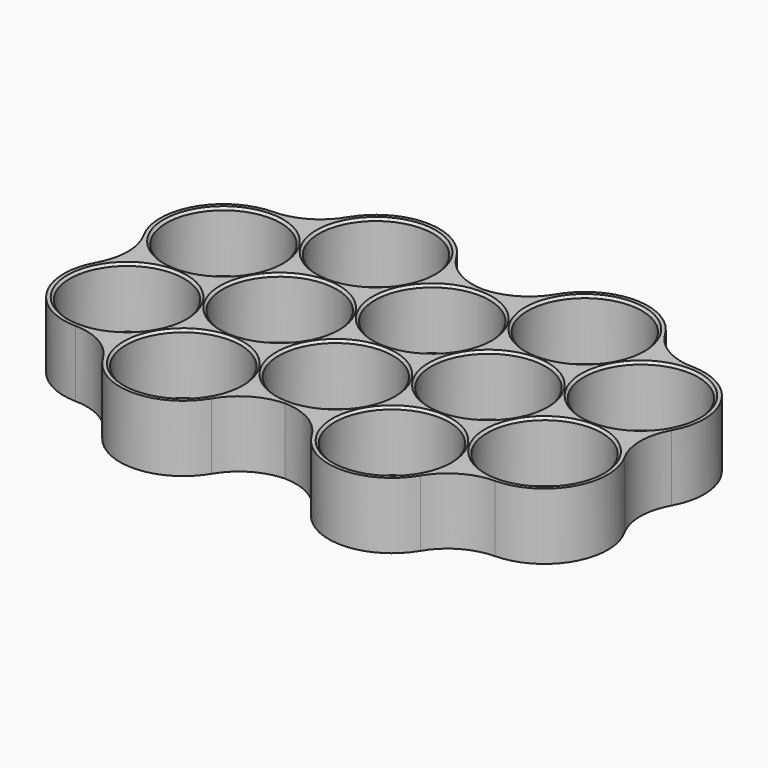
from build123d import *

# Parameters (mm, degrees)
F0_R        = 9.5
F1_DEPTH    = 11
F0_R_2      = 6
F2_DEPTH    = 1
F3_T1_DEPTH = 11
F4_SIZE     = 0.4


# Not quite as in the source:
# - a fillet or chamfer that OpenCascade refuses, or shapes differently, is made with other operations: its cross-section is extruded or revolved along the edge and cut away or added


with BuildPart() as f1:
    # F0 (on Top) → F1 (new body)
    with BuildSketch(Plane.XY):
        with BuildLine():
            ThreePointArc((10.2610350972, 17.7726341266), (0, 30.5), (-10.2610350972, 17.7726341266))
            ThreePointArc((-10.2610350972, 17.7726341266), (-26.4137748154, 15.25), (-20.5220701944, 0))
            ThreePointArc((-20.5220701944, 0), (-26.4137748154, -15.25), (-10.2610350972, -17.7726341266))
            ThreePointArc((-10.2610350972, -17.7726341266), (0, -30.5), (10.2610350972, -17.7726341266))
            ThreePointArc((10.2610350972, -17.7726341266), (17.3205080757, -20.5), (24.3799810542, -17.7726341266))
            ThreePointArc((24.3799810542, -17.7726341266), (34.6410161514, -30.5), (44.9020512486, -17.7726341266))
            ThreePointArc((44.9020512486, -17.7726341266), (61.0547909668, -15.25), (55.1630863458, 0))
            ThreePointArc((55.1630863458, 0), (61.0547909668, 15.25), (44.9020512486, 17.7726341266))
            ThreePointArc((44.9020512486, 17.7726341266), (34.6410161514, 30.5), (24.3799810542, 17.7726341266))
            ThreePointArc((24.3799810542, 17.7726341266), (17.3205080757, 20.5), (10.2610350972, 17.7726341266))
        make_face()
        with Locations((0, -20)):
            Circle(F0_R, mode=Mode.SUBTRACT)
        with Locations((-17.3205080757, -10)):
            Circle(F0_R, mode=Mode.SUBTRACT)
        with Locations((34.6410161514, -20)):
            Circle(F0_R, mode=Mode.SUBTRACT)
        with Locations((17.3205080757, -10)):
            Circle(F0_R, mode=Mode.SUBTRACT)
        with Locations((51.9615242271, -10)):
            Circle(F0_R, mode=Mode.SUBTRACT)
        with Locations((-17.3205080757, 10)):
            Circle(F0_R, mode=Mode.SUBTRACT)
        Circle(F0_R, mode=Mode.SUBTRACT)
        with Locations((0, 20)):
            Circle(F0_R, mode=Mode.SUBTRACT)
        with Locations((34.6410161514, 0)):
            Circle(F0_R, mode=Mode.SUBTRACT)
        with Locations((17.3205080757, 10)):
            Circle(F0_R, mode=Mode.SUBTRACT)
        with Locations((51.9615242271, 10)):
            Circle(F0_R, mode=Mode.SUBTRACT)
        with Locations((34.6410161514, 20)):
            Circle(F0_R, mode=Mode.SUBTRACT)
    extrude(amount=F1_DEPTH)

    # F0 (on Top) → F2 (join)
    with BuildSketch(Plane.XY):
        with Locations((0, 20)):
            Circle(F0_R)
        with Locations((0, 20)):
            Circle(F0_R_2, mode=Mode.SUBTRACT)
        with Locations((-17.3205080757, 10)):
            Circle(F0_R)
        with Locations((-17.3205080757, 10)):
            Circle(F0_R_2, mode=Mode.SUBTRACT)
        with Locations((-17.3205080757, -10)):
            Circle(F0_R)
        with Locations((-17.3205080757, -10)):
            Circle(F0_R_2, mode=Mode.SUBTRACT)
        Circle(F0_R)
        Circle(F0_R_2, mode=Mode.SUBTRACT)
        with Locations((0, -20)):
            Circle(F0_R)
        with Locations((0, -20)):
            Circle(F0_R_2, mode=Mode.SUBTRACT)
        with Locations((17.3205080757, -10)):
            Circle(F0_R)
        with Locations((17.3205080757, -10)):
            Circle(F0_R_2, mode=Mode.SUBTRACT)
        with Locations((17.3205080757, 10)):
            Circle(F0_R)
        with Locations((17.3205080757, 10)):
            Circle(F0_R_2, mode=Mode.SUBTRACT)
        with Locations((34.6410161514, 20)):
            Circle(F0_R)
        with Locations((34.6410161514, 20)):
            Circle(F0_R_2, mode=Mode.SUBTRACT)
        with Locations((34.6410161514, 0)):
            Circle(F0_R)
        with Locations((34.6410161514, 0)):
            Circle(F0_R_2, mode=Mode.SUBTRACT)
        with Locations((34.6410161514, -20)):
            Circle(F0_R)
        with Locations((34.6410161514, -20)):
            Circle(F0_R_2, mode=Mode.SUBTRACT)
        with Locations((51.9615242271, -10)):
            Circle(F0_R)
        with Locations((51.9615242271, -10)):
            Circle(F0_R_2, mode=Mode.SUBTRACT)
        with Locations((51.9615242271, 10)):
            Circle(F0_R)
        with Locations((51.9615242271, 10)):
            Circle(F0_R_2, mode=Mode.SUBTRACT)
    extrude(amount=F2_DEPTH)

    # F3: fillet of radius 10 on 10 edges, made by hand

    # F3_s2 → F3_t1 (join)
    with BuildSketch(Plane.XY):
        with BuildLine():
            ThreePointArc((25.6222746499, 25.3770160619), (22.0329970294, 21.837729702), (17.1732463203, 20.4989672814))
            ThreePointArc((17.1732463203, 20.4989672814), (21.0357320415, 19.8207489981), (24.3799810542, 17.7726341266))
            ThreePointArc((24.3799810542, 17.7726341266), (24.2783860519, 21.692896164), (25.6222746499, 25.3770160619))
        make_face()
        with BuildLine():
            ThreePointArc((17.4677698311, 20.4989672814), (12.6080191219, 21.837729702), (9.0187415015, 25.3770160619))
            ThreePointArc((9.0187415015, 25.3770160619), (10.3626300995, 21.692896164), (10.2610350972, 17.7726341266))
            ThreePointArc((10.2610350972, 17.7726341266), (13.6052841099, 19.8207489981), (17.4677698311, 20.4989672814))
        make_face()
        with BuildLine():
            ThreePointArc((-9.0187415015, 25.3770160619), (-12.6080191219, 21.837729702), (-17.4677698311, 20.4989672814))
            ThreePointArc((-17.4677698311, 20.4989672814), (-13.6052841099, 19.8207489981), (-10.2610350972, 17.7726341266))
            ThreePointArc((-10.2610350972, 17.7726341266), (-10.3626300995, 21.692896164), (-9.0187415015, 25.3770160619))
        make_face()
        with BuildLine():
            ThreePointArc((-26.4865113326, 4.8780487805), (-25.2160382439, 0), (-26.4865113326, -4.8780487805))
            ThreePointArc((-26.4865113326, -4.8780487805), (-23.9679142094, -1.8721471658), (-20.5220701944, 0))
            ThreePointArc((-20.5220701944, 0), (-23.9679142094, 1.8721471658), (-26.4865113326, 4.8780487805))
        make_face()
        with BuildLine():
            ThreePointArc((-17.4677698311, -20.4989672814), (-12.6080191219, -21.837729702), (-9.0187415015, -25.3770160619))
            ThreePointArc((-9.0187415015, -25.3770160619), (-10.3626300995, -21.692896164), (-10.2610350972, -17.7726341266))
            ThreePointArc((-10.2610350972, -17.7726341266), (-13.6052841099, -19.8207489981), (-17.4677698311, -20.4989672814))
        make_face()
        with BuildLine():
            ThreePointArc((9.0187415015, -25.3770160619), (12.6080191219, -21.837729702), (17.4677698311, -20.4989672814))
            ThreePointArc((17.4677698311, -20.4989672814), (13.6052841099, -19.8207489981), (10.2610350972, -17.7726341266))
            ThreePointArc((10.2610350972, -17.7726341266), (10.3626300995, -21.692896164), (9.0187415015, -25.3770160619))
        make_face()
        with BuildLine():
            ThreePointArc((25.6222746499, -25.3770160619), (22.0329970294, -21.837729702), (17.1732463203, -20.4989672814))
            ThreePointArc((17.1732463203, -20.4989672814), (21.0357320415, -19.8207489981), (24.3799810542, -17.7726341266))
            ThreePointArc((24.3799810542, -17.7726341266), (24.2783860519, -21.692896164), (25.6222746499, -25.3770160619))
        make_face()
        with BuildLine():
            ThreePointArc((52.1087859825, -20.4989672814), (47.2490352733, -21.837729702), (43.6597576529, -25.3770160619))
            ThreePointArc((43.6597576529, -25.3770160619), (45.0036462508, -21.692896164), (44.9020512486, -17.7726341266))
            ThreePointArc((44.9020512486, -17.7726341266), (48.2463002613, -19.8207489981), (52.1087859825, -20.4989672814))
        make_face()
        with BuildLine():
            ThreePointArc((61.1275274839, 4.8780487805), (59.8570543952, 0), (61.1275274839, -4.8780487805))
            ThreePointArc((61.1275274839, -4.8780487805), (58.6089303607, -1.8721471658), (55.1630863458, 0))
            ThreePointArc((55.1630863458, 0), (58.6089303607, 1.8721471658), (61.1275274839, 4.8780487805))
        make_face()
        with BuildLine():
            ThreePointArc((52.1087859825, 20.4989672814), (47.2490352733, 21.837729702), (43.6597576529, 25.3770160619))
            ThreePointArc((43.6597576529, 25.3770160619), (45.0036462508, 21.692896164), (44.9020512486, 17.7726341266))
            ThreePointArc((44.9020512486, 17.7726341266), (48.2463002613, 19.8207489981), (52.1087859825, 20.4989672814))
        make_face()
    extrude(amount=F3_T1_DEPTH)

    # F4
    f4_edges = [f1.edges().sort_by_distance(p)[0] for p in [
        (-26.820508, 10, 11),
        (-9.5, 20, 11),
        (-26.820508, -10, 11),
        (-9.5, 0, 11),
        (-9.5, -20, 11),
        (7.820508, -10, 11),
        (7.820508, 10, 11),
        (25.141016, 20, 11),
        (25.141016, 0, 11),
        (42.461524, 10, 11),
        (42.461524, -10, 11),
        (25.141016, -20, 11),
    ]]
    chamfer(f4_edges, length=F4_SIZE)


solid = f1.part
